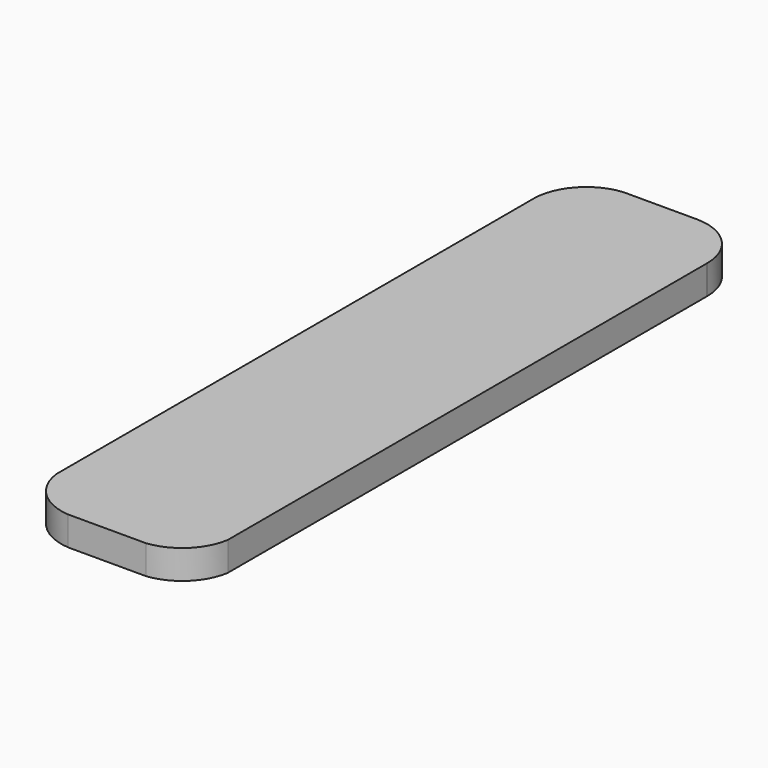
from build123d import *

# Parameters (mm, degrees)
F0_R          = 1.25
F0_R_2        = 12
F1_DEPTH      = 5
F0_R_3        = 1
F2_START      = 3
F0_R_4        = 2
F2_DEPTH      = 2
F4_START      = 1.6
F4_DEPTH      = 3.4
F5_DEPTH      = 1.3
F5_DEPTH_BACK = 0.1


# Not quite as in the source:
# - a feature of the source that left no trace in its solid (it failed there, or was rolled back) is left out


with BuildPart() as f1:
    # F0 (on Top) → F1 (new body)
    with BuildSketch(Plane.XY):
        with BuildLine():
            Line((6.0037070689, 60.0215111673), (-5, 60.0215111673))
            Line((-5, 60.0215111673), (-6.7870675903, 60.0215111673))
            ThreePointArc((-6.7870675903, 60.0215111673), (-12.5859769766, 57.1353808627), (-15, 51.1245913098))
            Line((-15, 51.1245913098), (-15, 50.7903024554))
            Line((-15, 50.7903024554), (-15, -49.5038591325))
            Line((-15, -49.5038591325), (-15, -51.7690908138))
            ThreePointArc((-15, -51.7690908138), (-12.1695256151, -57.4125609321), (-6.4009595691, -59.9784888327))
            Line((-6.4009595691, -59.9784888327), (-5, -59.9784888327))
            Line((-5, -59.9784888327), (5, -59.9784888327))
            Line((5, -59.9784888327), (7.0074141379, -59.9784888327))
            ThreePointArc((7.0074141379, -59.9784888327), (12.2930504345, -57.5138166091), (15, -52.3480655233))
            Line((15, -52.3480655233), (15, -49.5038591325))
            Line((15, -49.5038591325), (15, 50.7903024554))
            Line((15, 50.7903024554), (15, 50.95497525))
            ThreePointArc((15, 50.95497525), (12.3454627339, 57.317569046), (6.0037070689, 60.0215111673))
        make_face()
        with Locations((-9.525, -56.2587864697)):
            Circle(F0_R, mode=Mode.SUBTRACT)
        with Locations((-9.525, -30.4671674967)):
            Circle(F0_R, mode=Mode.SUBTRACT)
        with Locations((0, -44.7514858243)):
            Circle(F0_R_2, mode=Mode.SUBTRACT)
        with Locations((-9.525, 0)):
            Circle(F0_R, mode=Mode.SUBTRACT)
        with Locations((0, -15.4157546586)):
            Circle(F0_R_2, mode=Mode.SUBTRACT)
        with Locations((9.525, -56.2587864697)):
            Circle(F0_R, mode=Mode.SUBTRACT)
        with Locations((9.525, -30.4671674967)):
            Circle(F0_R, mode=Mode.SUBTRACT)
        with Locations((9.525, 0)):
            Circle(F0_R, mode=Mode.SUBTRACT)
        with Locations((-9.525, 29.1974432766)):
            Circle(F0_R, mode=Mode.SUBTRACT)
        with Locations((0, 15.3948861798)):
            Circle(F0_R_2, mode=Mode.SUBTRACT)
        with Locations((-9.525, 55.7628124952)):
            Circle(F0_R, mode=Mode.SUBTRACT)
        with Locations((0, 44.3624239764)):
            Circle(F0_R_2, mode=Mode.SUBTRACT)
        with Locations((9.525, 29.1974432766)):
            Circle(F0_R, mode=Mode.SUBTRACT)
        with Locations((9.525, 55.7628124952)):
            Circle(F0_R, mode=Mode.SUBTRACT)
        with BuildLine():
            ThreePointArc((15, 50.7903024554), (15.0003704536, 50.8726388527), (15, 50.95497525))
            Line((15, 50.95497525), (15, 50.7903024554))
        make_face()
    extrude(amount=F1_DEPTH)



with BuildPart() as f1b:
    # F0 (on Top) → F1, piece 2 (new body)
    with BuildSketch(Plane.XY):
        with Locations((-9.525, 44.3624239764)):
            Circle(F0_R_3)
    extrude(amount=F1_DEPTH)


with BuildPart() as f1c:
    # F0 (on Top) → F1, piece 3 (new body)
    with BuildSketch(Plane.XY):
        with Locations((9.525, 44.3624239764)):
            Circle(F0_R_3)
    extrude(amount=F1_DEPTH)


with BuildPart() as f1d:
    # F0 (on Top) → F1, piece 4 (new body)
    with BuildSketch(Plane.XY):
        with Locations((9.525, 15.3948861798)):
            Circle(F0_R_3)
    extrude(amount=F1_DEPTH)


with BuildPart() as f1e:
    # F0 (on Top) → F1, piece 5 (new body)
    with BuildSketch(Plane.XY):
        with Locations((-9.525, 15.3948861798)):
            Circle(F0_R_3)
    extrude(amount=F1_DEPTH)


with BuildPart() as f1f:
    # F0 (on Top) → F1, piece 6 (new body)
    with BuildSketch(Plane.XY):
        with Locations((9.525, -15.4157546586)):
            Circle(F0_R_3)
    extrude(amount=F1_DEPTH)


with BuildPart() as f1g:
    # F0 (on Top) → F1, piece 7 (new body)
    with BuildSketch(Plane.XY):
        with Locations((-9.525, -15.4157546586)):
            Circle(F0_R_3)
    extrude(amount=F1_DEPTH)


with BuildPart() as f1h:
    # F0 (on Top) → F1, piece 8 (new body)
    with BuildSketch(Plane.XY):
        with Locations((9.525, -44.7514858243)):
            Circle(F0_R_3)
    extrude(amount=F1_DEPTH)


with BuildPart() as f1i:
    # F0 (on Top) → F1, piece 9 (new body)
    with BuildSketch(Plane.XY):
        with Locations((-9.525, -44.7514858243)):
            Circle(F0_R_3)
    extrude(amount=F1_DEPTH)


with BuildPart() as f1_1:
    add(f1.part)

    add(f1b.part)  # F2 merges F1b

    add(f1c.part)  # F2 merges F1c

    add(f1d.part)  # F2 merges F1d

    add(f1e.part)  # F2 merges F1e

    add(f1f.part)  # F2 merges F1f

    add(f1g.part)  # F2 merges F1g

    add(f1h.part)  # F2 merges F1h

    add(f1i.part)  # F2 merges F1i
    # F0 (on Top) → F2 (join)
    with BuildSketch(Plane.XY.offset(F2_START)):
        with Locations((0, 44.3624239764)):
            Circle(F0_R_2)
        with Locations((-9.525, 44.3624239764)):
            Circle(F0_R_4, mode=Mode.SUBTRACT)
        with Locations((9.525, 44.3624239764)):
            Circle(F0_R_4, mode=Mode.SUBTRACT)
        with Locations((0, 15.3948861798)):
            Circle(F0_R_2)
        with Locations((-9.525, 15.3948861798)):
            Circle(F0_R_4, mode=Mode.SUBTRACT)
        with Locations((9.525, 15.3948861798)):
            Circle(F0_R_4, mode=Mode.SUBTRACT)
        with Locations((0, -15.4157546586)):
            Circle(F0_R_2)
        with Locations((-9.525, -15.4157546586)):
            Circle(F0_R_4, mode=Mode.SUBTRACT)
        with Locations((9.525, -15.4157546586)):
            Circle(F0_R_4, mode=Mode.SUBTRACT)
        with Locations((0, -44.7514858243)):
            Circle(F0_R_2)
        with Locations((-9.525, -44.7514858243)):
            Circle(F0_R_4, mode=Mode.SUBTRACT)
        with Locations((9.525, -44.7514858243)):
            Circle(F0_R_4, mode=Mode.SUBTRACT)
        with Locations((9.525, 44.3624239764)):
            Circle(F0_R_4)
        with Locations((9.525, 44.3624239764)):
            Circle(F0_R_3, mode=Mode.SUBTRACT)
        with Locations((-9.525, 44.3624239764)):
            Circle(F0_R_4)
        with Locations((-9.525, 44.3624239764)):
            Circle(F0_R_3, mode=Mode.SUBTRACT)
        with Locations((9.525, 15.3948861798)):
            Circle(F0_R_4)
        with Locations((9.525, 15.3948861798)):
            Circle(F0_R_3, mode=Mode.SUBTRACT)
        with Locations((-9.525, 15.3948861798)):
            Circle(F0_R_4)
        with Locations((-9.525, 15.3948861798)):
            Circle(F0_R_3, mode=Mode.SUBTRACT)
        with Locations((9.525, -15.4157546586)):
            Circle(F0_R_4)
        with Locations((9.525, -15.4157546586)):
            Circle(F0_R_3, mode=Mode.SUBTRACT)
        with Locations((-9.525, -15.4157546586)):
            Circle(F0_R_4)
        with Locations((-9.525, -15.4157546586)):
            Circle(F0_R_3, mode=Mode.SUBTRACT)
        with Locations((9.525, -44.7514858243)):
            Circle(F0_R_4)
        with Locations((9.525, -44.7514858243)):
            Circle(F0_R_3, mode=Mode.SUBTRACT)
        with Locations((-9.525, -44.7514858243)):
            Circle(F0_R_4)
        with Locations((-9.525, -44.7514858243)):
            Circle(F0_R_3, mode=Mode.SUBTRACT)
        with Locations((9.525, -56.2587864697)):
            Circle(F0_R)
        with Locations((-9.525, -56.2587864697)):
            Circle(F0_R)
        with Locations((-9.525, -30.4671674967)):
            Circle(F0_R)
        with Locations((9.525, -30.4671674967)):
            Circle(F0_R)
        with Locations((9.525, 0)):
            Circle(F0_R)
        with Locations((-9.525, 0)):
            Circle(F0_R)
        with Locations((-9.525, 29.1974432766)):
            Circle(F0_R)
        with Locations((9.525, 29.1974432766)):
            Circle(F0_R)
        with Locations((-9.525, 55.7628124952)):
            Circle(F0_R)
        with Locations((9.525, 55.7628124952)):
            Circle(F0_R)
        with Locations((9.525, 44.3624239764)):
            Circle(F0_R_3)
        with Locations((-9.525, 44.3624239764)):
            Circle(F0_R_3)
        with Locations((9.525, 15.3948861798)):
            Circle(F0_R_3)
        with Locations((-9.525, 15.3948861798)):
            Circle(F0_R_3)
        with Locations((9.525, -15.4157546586)):
            Circle(F0_R_3)
        with Locations((-9.525, -15.4157546586)):
            Circle(F0_R_3)
        with Locations((9.525, -44.7514858243)):
            Circle(F0_R_3)
        with Locations((-9.525, -44.7514858243)):
            Circle(F0_R_3)
    extrude(amount=F2_DEPTH)

    # F0 (on Top) → F4 (join)
    with BuildSketch(Plane.XY.offset(F4_START)):
        with Locations((9.525, 44.3624239764)):
            Circle(F0_R_4)
        with Locations((9.525, 44.3624239764)):
            Circle(F0_R_3, mode=Mode.SUBTRACT)
        with Locations((-9.525, 44.3624239764)):
            Circle(F0_R_4)
        with Locations((-9.525, 44.3624239764)):
            Circle(F0_R_3, mode=Mode.SUBTRACT)
        with Locations((9.525, 15.3948861798)):
            Circle(F0_R_4)
        with Locations((9.525, 15.3948861798)):
            Circle(F0_R_3, mode=Mode.SUBTRACT)
        with Locations((-9.525, 15.3948861798)):
            Circle(F0_R_4)
        with Locations((-9.525, 15.3948861798)):
            Circle(F0_R_3, mode=Mode.SUBTRACT)
        with Locations((9.525, -15.4157546586)):
            Circle(F0_R_4)
        with Locations((9.525, -15.4157546586)):
            Circle(F0_R_3, mode=Mode.SUBTRACT)
        with Locations((-9.525, -15.4157546586)):
            Circle(F0_R_4)
        with Locations((-9.525, -15.4157546586)):
            Circle(F0_R_3, mode=Mode.SUBTRACT)
        with Locations((9.525, -44.7514858243)):
            Circle(F0_R_4)
        with Locations((9.525, -44.7514858243)):
            Circle(F0_R_3, mode=Mode.SUBTRACT)
        with Locations((-9.525, -44.7514858243)):
            Circle(F0_R_4)
        with Locations((-9.525, -44.7514858243)):
            Circle(F0_R_3, mode=Mode.SUBTRACT)
    extrude(amount=F4_DEPTH)

    # F0 (on Top) → F5 (cut, two sides)
    with BuildSketch(Plane.XY) as f5_sk:
        with Locations((9.525, -56.2587864697)):
            Circle(F0_R)
        with Locations((-9.525, -56.2587864697)):
            Circle(F0_R)
        with Locations((-9.525, -30.4671674967)):
            Circle(F0_R)
        with Locations((9.525, -30.4671674967)):
            Circle(F0_R)
        with Locations((9.525, 0)):
            Circle(F0_R)
        with Locations((-9.525, 0)):
            Circle(F0_R)
        with Locations((9.525, 29.1974432766)):
            Circle(F0_R)
        with Locations((-9.525, 29.1974432766)):
            Circle(F0_R)
        with Locations((9.525, 55.7628124952)):
            Circle(F0_R)
        with Locations((-9.525, 55.7628124952)):
            Circle(F0_R)
    extrude(amount=F5_DEPTH, mode=Mode.SUBTRACT)
    extrude(f5_sk.sketch, amount=-F5_DEPTH_BACK, mode=Mode.SUBTRACT)


solid = f1_1.part
